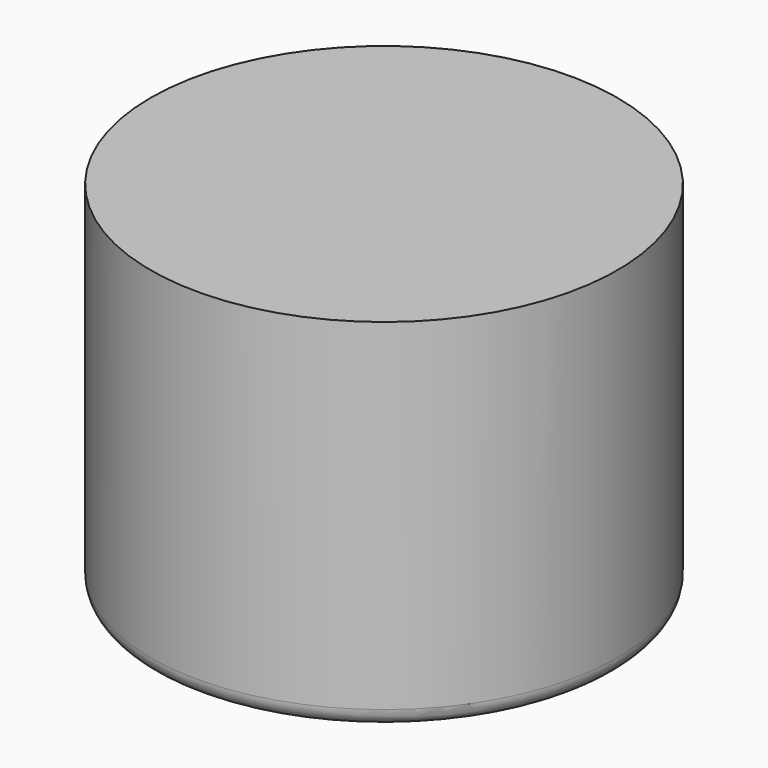
from build123d import *

# Parameters (mm, degrees)
F2_R = 0.5
F3_R = 0.99999


# Not quite as in the source:
# - a fillet or chamfer is up to 0.001 mm smaller than in the source, because OpenCascade refuses the exact size


with BuildPart() as f1:
    # F0 (on Front) → F1 (revolve)
    with BuildSketch(Plane.XZ):
        Polygon((31.5384635292, 12.9299255153), (18.5384635292, 12.9299255153), (18.5384635292, -7.0700744847), (20.5384635292, -7.0700744847), (20.5384635292, 10.9299255153), (31.5384635292, 10.9299255153), align=None)
    revolve(axis=Axis((31.5384635292, 0, 11.9299255153), (0, 0, -1)))

    # F2
    f2_edges = [f1.edges().sort_by_distance(p)[0] for p in [
        (42.538464, 0, 10.929926),
    ]]
    fillet(f2_edges, radius=F2_R)

    # F3 (radius 1 in the source; OpenCascade refuses exactly that, so slightly less here)
    f3_edges = [f1.edges().sort_by_distance(p)[0] for p in [
        (44.538464, 0, -7.070074),
        (42.538464, 0, -7.070074),
    ]]
    fillet(f3_edges, radius=F3_R)


solid = f1.part
